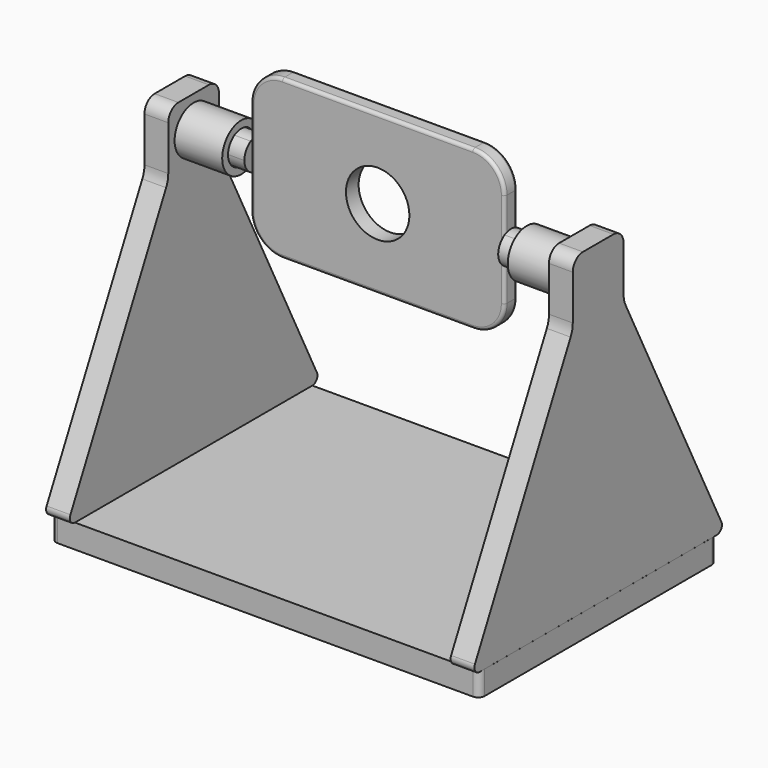
from build123d import *

# Parameters (mm, degrees)
F0_W      = 50.8
F0_H      = 31.75
F0_R      = 6.35
F1_DEPTH  = 3.175
F3_DEPTH  = 12.7
F5_DEPTH  = 12.7
F6_R      = 6.35
F7_R      = 0.635
F8_R      = 0.635
F9_R      = 0.635
F9_2_R    = 0.635
F10_R     = 4.7625
F10_R_2   = 3.302
F11_DEPTH = 9.525
F12_R     = 4.7625
F12_R_2   = 3.302
F13_DEPTH = 9.525
F14_W     = 12.7
F14_H     = 12.7
F14_R     = 4.7625
F14_R_2   = 3.302
F15_DEPTH = 4.7625
F16_W     = 12.7
F16_H     = 12.7
F16_R     = 4.7625
F16_R_2   = 3.302
F17_DEPTH = 4.7625
F18_R     = 2.54
F18_2_R   = 2.54
F19_R     = 5.08
F19_2_R   = 5.08
F20_R     = 1.27
F20_2_R   = 1.27
F21_W     = 4.7625
F21_H     = 59.3842198926
F21_W_2   = 80.9674418151
F22_DEPTH = 4.7625
F23_R     = 1.27


# Not quite as in the source:
# - a feature names something its author has since deleted; it is built from what else it names


with BuildPart() as f1:
    # F0 (on Front) → F1 (new body)
    with BuildSketch(Plane.XZ):
        with Locations((-12.7, 0)):
            Rectangle(F0_W, F0_H)
        with Locations((-12.7, 0)):
            Circle(F0_R, mode=Mode.SUBTRACT)
    extrude(amount=F1_DEPTH)

    # F6
    f6_edges = [f1.edges().sort_by_distance(p)[0] for p in [
        (-38.1, -1.5875, 15.875),
        (-38.1, -1.5875, -15.875),
        (12.7, -1.5875, -15.875),
        (12.7, -1.5875, 15.875),
    ]]
    fillet(f6_edges, radius=F6_R)

    # F7
    f7_edges = [f1.edges().sort_by_distance(p)[0] for p in [
        (-12.7, -3.175, 15.875),
    ]]
    fillet(f7_edges, radius=F7_R)

    # F8
    f8_edges = [f1.edges().sort_by_distance(p)[0] for p in [
        (-12.7, 0, 15.875),
    ]]
    fillet(f8_edges, radius=F8_R)


with BuildPart() as f3:
    # F2 (on face) → F3 (new body)
    with BuildSketch(Plane(origin=(-38.1, 0, 0), x_dir=(0, -1, 0), z_dir=(-1, 0, 0))):
        with BuildLine():
            Line((0, -2.749630657), (0, 2.749630657))
            ThreePointArc((0, 2.749630657), (-1.5875, 0), (0, -2.749630657))
        make_face()
        with BuildLine():
            Line((3.175, -2.749630657), (3.175, 2.749630657))
            ThreePointArc((3.175, 2.749630657), (1.5875, 3.175), (0, 2.749630657))
            Line((0, 2.749630657), (0, -2.749630657))
            ThreePointArc((0, -2.749630657), (1.5875, -3.175), (3.175, -2.749630657))
        make_face()
        with BuildLine():
            ThreePointArc((3.175, -2.749630657), (4.337130657, -1.5875), (4.7625, 0))
            ThreePointArc((4.7625, 0), (4.337130657, 1.5875), (3.175, 2.749630657))
            Line((3.175, 2.749630657), (3.175, -2.749630657))
        make_face()
    extrude(amount=F3_DEPTH)

    # F9
    f9_edges = [f3.edges().sort_by_distance(p)[0] for p in [
        (-50.8, 0, 2.749631),
    ]]
    fillet(f9_edges, radius=F9_R)


with BuildPart() as f5:
    # F4 (on face) → F5 (new body)
    with BuildSketch(Plane.YZ.offset(12.7)):
        with BuildLine():
            Line((0, -2.749630657), (0, 2.749630657))
            ThreePointArc((0, 2.749630657), (-1.5875, 3.175), (-3.175, 2.749630657))
            Line((-3.175, 2.749630657), (-3.175, -2.749630657))
            ThreePointArc((-3.175, -2.749630657), (-1.5875, -3.175), (0, -2.749630657))
        make_face()
        with BuildLine():
            Line((-3.175, -2.749630657), (-3.175, 2.749630657))
            ThreePointArc((-3.175, 2.749630657), (-4.7625, 0), (-3.175, -2.749630657))
        make_face()
        with BuildLine():
            ThreePointArc((0, -2.749630657), (1.162130657, -1.5875), (1.5875, 0))
            ThreePointArc((1.5875, 0), (1.162130657, 1.5875), (0, 2.749630657))
            Line((0, 2.749630657), (0, -2.749630657))
        make_face()
    extrude(amount=F5_DEPTH)

    # F9#2
    f9_2_edges = [f5.edges().sort_by_distance(p)[0] for p in [
        (25.4, -3.175, 2.749631),
    ]]
    fillet(f9_2_edges, radius=F9_2_R)


with BuildPart() as f11:
    # F10 (on face) → F11 (new body)
    with BuildSketch(Plane.YZ.offset(25.4)):
        with Locations((-1.5875, 0)):
            Circle(F10_R)
        with Locations((-1.5875, 0)):
            Circle(F10_R_2, mode=Mode.SUBTRACT)
    extrude(amount=-F11_DEPTH)


with BuildPart() as f13:
    # F12 (on face) → F13 (new body)
    with BuildSketch(Plane(origin=(-50.8, 0, 0), x_dir=(0, -1, 0), z_dir=(-1, 0, 0))):
        with Locations((1.5875, 0)):
            Circle(F12_R)
        with Locations((1.5875, 0)):
            Circle(F12_R_2, mode=Mode.SUBTRACT)
    extrude(amount=-F13_DEPTH)


with BuildPart() as f15:
    # F14 (on face) → F15 (new body)
    with BuildSketch(Plane.YZ.offset(25.4)):
        with Locations((-1.5875, 0)):
            Rectangle(F14_W, F14_H)
        with Locations((-1.5875, 0)):
            Circle(F14_R, mode=Mode.SUBTRACT)
        with Locations((-1.5875, 0)):
            Circle(F14_R)
        with Locations((-1.5875, 0)):
            Circle(F14_R_2, mode=Mode.SUBTRACT)
        with Locations((-1.5875, 0)):
            Circle(F14_R_2)
        Polygon((30.1625, -57.15), (4.7625, -6.35), (-7.9375, -6.35), (-33.3375, -57.15), align=None)
    extrude(amount=F15_DEPTH)

    # F18#2
    f18_2_edges = [f15.edges().sort_by_distance(p)[0] for p in [
        (27.78125, -7.9375, 6.35),
        (27.78125, 4.7625, 6.35),
    ]]
    fillet(f18_2_edges, radius=F18_2_R)

    # F19#2
    f19_2_edges = [f15.edges().sort_by_distance(p)[0] for p in [
        (27.78125, -7.9375, -6.35),
        (27.78125, 4.7625, -6.35),
    ]]
    fillet(f19_2_edges, radius=F19_2_R)

    # F20#2
    f20_2_edges = [f15.edges().sort_by_distance(p)[0] for p in [
        (27.78125, -33.3375, -57.15),
        (27.78125, 30.1625, -57.15),
    ]]
    fillet(f20_2_edges, radius=F20_2_R)


with BuildPart() as f17:
    # F16 (on face) → F17 (new body)
    with BuildSketch(Plane(origin=(-50.8, 0, 0), x_dir=(0, -1, 0), z_dir=(-1, 0, 0))):
        with Locations((1.5875, 0)):
            Rectangle(F16_W, F16_H)
        with Locations((1.5875, 0)):
            Circle(F16_R, mode=Mode.SUBTRACT)
        with Locations((1.5875, 0)):
            Circle(F16_R)
        with Locations((1.5875, 0)):
            Circle(F16_R_2, mode=Mode.SUBTRACT)
        with Locations((1.5875, 0)):
            Circle(F16_R_2)
        Polygon((33.3375, -57.15), (7.9375, -6.35), (-4.7625, -6.35), (-30.1625, -57.15), align=None)
    extrude(amount=F17_DEPTH)

    # F18
    f18_edges = [f17.edges().sort_by_distance(p)[0] for p in [
        (-53.18125, -7.9375, 6.35),
        (-53.18125, 4.7625, 6.35),
    ]]
    fillet(f18_edges, radius=F18_R)

    # F19
    f19_edges = [f17.edges().sort_by_distance(p)[0] for p in [
        (-53.18125, -7.9375, -6.35),
        (-53.18125, 4.7625, -6.35),
    ]]
    fillet(f19_edges, radius=F19_R)

    # F20
    f20_edges = [f17.edges().sort_by_distance(p)[0] for p in [
        (-53.18125, -33.3375, -57.15),
        (-53.18125, 30.1625, -57.15),
    ]]
    fillet(f20_edges, radius=F20_R)


with BuildPart() as f22:
    # F21 (on face) → F22 (new body)
    with BuildSketch(Plane(origin=(0, 0, -57.15), x_dir=(1, 0, 0), z_dir=(0, 0, -1))):
        with Locations((-53.18125, 1.590486888)):
            Rectangle(F21_W, F21_H)
        with Locations((-10.3162790924, 1.590486888)):
            Rectangle(F21_W_2, F21_H)
    extrude(amount=F22_DEPTH)

    # F23
    f23_edges = [f22.edges().sort_by_distance(p)[0] for p in [
        (-55.5625, -31.282597, -59.53125),
        (-55.5625, 28.101623, -59.53125),
        (30.167442, 28.101623, -59.53125),
        (30.167442, -31.282597, -59.53125),
    ]]
    fillet(f23_edges, radius=F23_R)


solid = Compound([f1.part, f3.part, f5.part, f11.part, f13.part, f15.part, f17.part, f22.part])
